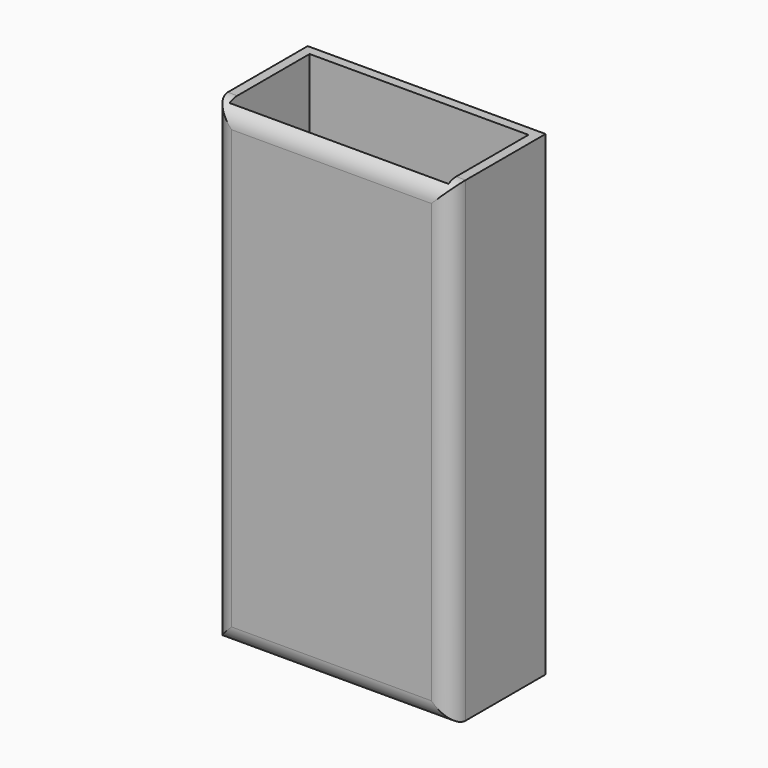
from build123d import *

# Parameters (mm, degrees)
F0_W        = 63.5
F0_H        = 127
F1_DEPTH    = 31.75
F2_T        = -2.54
F3_T1_DEPTH = 88.9
F3_T3_DEPTH = 152.4


# Not quite as in the source:
# - a fillet or chamfer that OpenCascade refuses, or shapes differently, is made with other operations: its cross-section is extruded or revolved along the edge and cut away or added


with BuildPart() as f1:
    # F0 (on Front) → F1 (new body)
    with BuildSketch(Plane.XZ):
        Rectangle(F0_W, F0_H)
    extrude(amount=F1_DEPTH)

    # F2
    f2_openings = [f1.faces().sort_by_distance(p)[0] for p in [
        (0, -15.875, 63.5),
    ]]
    offset(amount=F2_T, openings=f2_openings)

    # F3: fillet of radius 5.08 on 4 edges, made by hand

    # F3_s2 → F3_t1 (cut)
    with BuildSketch(Plane.YZ.offset(-44.45)):
        with BuildLine():
            ThreePointArc((-31.75, 58.42), (-30.2621024484, 62.0121024484), (-26.67, 63.5))
            Line((-26.67, 63.5), (-31.75, 63.5))
            Line((-31.75, 63.5), (-31.75, 58.42))
        make_face()
        with BuildLine():
            ThreePointArc((-26.67, -63.5), (-30.2621024484, -62.0121024484), (-31.75, -58.42))
            Line((-31.75, -58.42), (-31.75, -63.5))
            Line((-31.75, -63.5), (-26.67, -63.5))
        make_face()
    extrude(amount=F3_T1_DEPTH, mode=Mode.SUBTRACT)

    # F3_s4 → F3_t3 (cut)
    with BuildSketch(Plane.XY.offset(-76.2)):
        with BuildLine():
            ThreePointArc((-31.75, -26.67), (-30.2621024484, -30.2621024484), (-26.67, -31.75))
            Line((-26.67, -31.75), (-31.75, -31.75))
            Line((-31.75, -31.75), (-31.75, -26.67))
        make_face()
        with BuildLine():
            ThreePointArc((31.75, -26.67), (30.2621024484, -30.2621024484), (26.67, -31.75))
            Line((26.67, -31.75), (31.75, -31.75))
            Line((31.75, -31.75), (31.75, -26.67))
        make_face()
    extrude(amount=F3_T3_DEPTH, mode=Mode.SUBTRACT)


solid = f1.part
